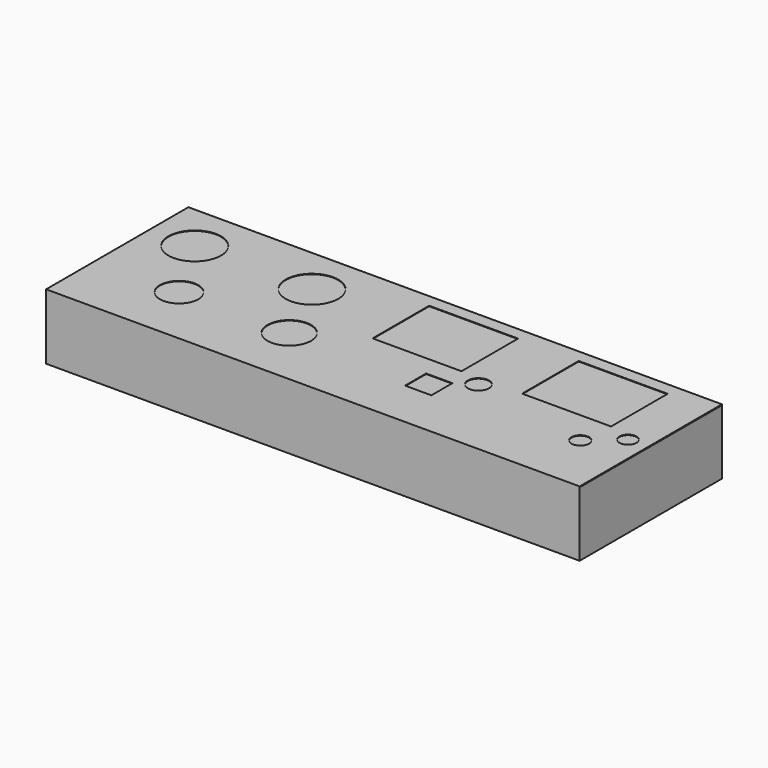
from build123d import *

# Parameters (mm, degrees)
F1_DEPTH = 209.55
F2_W     = 20.6375
F2_H     = 20.6375
F2_W_2   = 69.85
F2_H_2   = 55.5625
F3_DEPTH = 0.4064


# Not quite as in the source:
# - the dataset's text gives a spline's control points without its knots; the knots are read off the source's solid


with BuildPart() as f1:
    # F0 (on Right) → F1 (new body, symmetric)
    with BuildSketch(Plane.YZ):
        Polygon((-139.7, 0), (0, 0), (0, 50.8), (-139.2936, 50.8), (-139.2936, 51.054), (0, 51.054), (0, 51.4604), (-139.7, 51.4604), align=None)
    extrude(amount=F1_DEPTH, both=True)

    # F2 (on face) → F3 (cut, through all)
    with BuildSketch(Plane.XY.offset(51.4604)):
        with Locations((52.6280792475, -91.7013814436)):
            Rectangle(F2_W, F2_H)
        with Locations((139.9405792475, -37.7263814436)):
            Rectangle(F2_W_2, F2_H_2)
        with Locations((22.4655792475, -37.7263814436)):
            Rectangle(F2_W_2, F2_H_2)
        with BuildLine():
            add(Edge.make_bspline(
                [(-68.9765797525, -103.7685150436), (-65.8170737525, -106.9276908436), (-61.3770521525, -108.7670064436), (-56.9094207525, -108.7670064436), (-52.4415099525, -108.7670064436), (-48.0011327525, -106.9276908436), (-44.8419569525, -103.7685150436), (-41.6828065525, -100.6093646436), (-39.8437957525, -96.1693430436), (-39.8437957525, -91.7013814436), (-39.8437957525, -87.2334452436), (-41.6828065525, -82.7933728436), (-44.8419569525, -79.6342478436), (-48.0011327525, -76.4750974436), (-52.4415099525, -74.6357564436), (-56.9094207525, -74.6357564436)],
                knots=[3, 3, 3, 3, 4, 4, 4, 5, 5, 5, 6, 6, 6, 7, 7, 7, 8, 8, 8, 8], degree=3))
            add(Edge.make_bspline(
                [(-56.9094207525, -74.6357564436), (-61.3770521525, -74.6357564436), (-65.8170737525, -76.4750974436), (-68.9765797525, -79.6342478436)],
                knots=[0, 0, 0, 0, 1, 1, 1, 1], degree=3))
            add(Edge.make_bspline(
                [(-68.9765797525, -79.6342478436), (-72.1357047525, -82.7933728436), (-73.9750457525, -87.2334452436), (-73.9750457525, -91.7013814436), (-73.9750457525, -96.1693430436), (-72.1357047525, -100.6093646436), (-68.9765797525, -103.7685150436)],
                knots=[1, 1, 1, 1, 2, 2, 2, 3, 3, 3, 3], degree=3))
        make_face()
        with BuildLine():
            add(Edge.make_bspline(
                [(82.3340650475, -66.7578702436), (80.7910150475, -65.2151250436), (78.6226678475, -64.3170064436), (76.4405792475, -64.3170064436)],
                knots=[7, 7, 7, 7, 8, 8, 8, 8], degree=3))
            add(Edge.make_bspline(
                [(76.4405792475, -64.3170064436), (74.2587700475, -64.3170064436), (72.0901180475, -65.2151250436), (70.5473728475, -66.7578702436)],
                knots=[0, 0, 0, 0, 1, 1, 1, 1], degree=3))
            add(Edge.make_bspline(
                [(70.5473728475, -66.7578702436), (69.0046784475, -68.3009202436), (68.1062042475, -70.4695722436), (68.1062042475, -72.6513814436), (68.1062042475, -74.8331652436), (69.0046784475, -77.0018680436), (70.5473728475, -78.5445624436)],
                knots=[1, 1, 1, 1, 2, 2, 2, 3, 3, 3, 3], degree=3))
            add(Edge.make_bspline(
                [(70.5473728475, -78.5445624436), (72.0901180475, -80.0876124436), (74.2587700475, -80.9857564436), (76.4405792475, -80.9857564436), (78.6226678475, -80.9857564436), (80.7910150475, -80.0876124436), (82.3340650475, -78.5445624436)],
                knots=[3, 3, 3, 3, 4, 4, 4, 5, 5, 5, 5], degree=3))
            add(Edge.make_bspline(
                [(82.3340650475, -78.5445624436), (83.8771658475, -77.0018680436), (84.7749542475, -74.8331652436), (84.7749542475, -72.6513814436), (84.7749542475, -70.4695722436), (83.8771658475, -68.3009202436), (82.3340650475, -66.7578702436)],
                knots=[5, 5, 5, 5, 6, 6, 6, 7, 7, 7, 7], degree=3))
        make_face()
        with BuildLine():
            add(Edge.make_bspline(
                [(-67.7163587525, -23.1332940436), (-71.5366203525, -19.3130324436), (-76.9064851525, -17.0888814436), (-82.3094207525, -17.0888814436)],
                knots=[7, 7, 7, 7, 8, 8, 8, 8], degree=3))
            add(Edge.make_bspline(
                [(-82.3094207525, -17.0888814436), (-87.7120515525, -17.0888814436), (-93.0815607525, -19.3130324436), (-96.9021525525, -23.1332940436)],
                knots=[0, 0, 0, 0, 1, 1, 1, 1], degree=3))
            add(Edge.make_bspline(
                [(-96.9021525525, -23.1332940436), (-100.7227697525, -26.9539112436), (-102.9469207525, -32.3234458436), (-102.9469207525, -37.7263814436), (-102.9469207525, -43.1293170436), (-100.7227697525, -48.4988770436), (-96.9021525525, -52.3194434436)],
                knots=[1, 1, 1, 1, 2, 2, 2, 3, 3, 3, 3], degree=3))
            add(Edge.make_bspline(
                [(-96.9021525525, -52.3194434436), (-93.0815607525, -56.1397050436), (-87.7120515525, -58.3638814436), (-82.3094207525, -58.3638814436), (-76.9064851525, -58.3638814436), (-71.5366203525, -56.1397050436), (-67.7163587525, -52.3194434436)],
                knots=[3, 3, 3, 3, 4, 4, 4, 5, 5, 5, 5], degree=3))
            add(Edge.make_bspline(
                [(-67.7163587525, -52.3194434436), (-63.8960971525, -48.4988770436), (-61.6719207525, -43.1293170436), (-61.6719207525, -37.7263814436), (-61.6719207525, -32.3234458436), (-63.8960971525, -26.9539112436), (-67.7163587525, -23.1332940436)],
                knots=[5, 5, 5, 5, 6, 6, 6, 7, 7, 7, 7], degree=3))
        make_face()
        with BuildLine():
            add(Edge.make_bspline(
                [(-159.7913587525, -23.1332940436), (-163.6116203525, -19.3130324436), (-168.9814851525, -17.0888814436), (-174.3844207525, -17.0888814436)],
                knots=[7, 7, 7, 7, 8, 8, 8, 8], degree=3))
            add(Edge.make_bspline(
                [(-174.3844207525, -17.0888814436), (-179.7870515525, -17.0888814436), (-185.1565607525, -19.3130324436), (-188.9771525525, -23.1332940436)],
                knots=[0, 0, 0, 0, 1, 1, 1, 1], degree=3))
            add(Edge.make_bspline(
                [(-188.9771525525, -23.1332940436), (-192.7977697525, -26.9539112436), (-195.0219207525, -32.3234458436), (-195.0219207525, -37.7263814436), (-195.0219207525, -43.1293170436), (-192.7977697525, -48.4988770436), (-188.9771525525, -52.3194434436)],
                knots=[1, 1, 1, 1, 2, 2, 2, 3, 3, 3, 3], degree=3))
            add(Edge.make_bspline(
                [(-188.9771525525, -52.3194434436), (-185.1565607525, -56.1397050436), (-179.7870515525, -58.3638814436), (-174.3844207525, -58.3638814436), (-168.9814851525, -58.3638814436), (-163.6116203525, -56.1397050436), (-159.7913587525, -52.3194434436)],
                knots=[3, 3, 3, 3, 4, 4, 4, 5, 5, 5, 5], degree=3))
            add(Edge.make_bspline(
                [(-159.7913587525, -52.3194434436), (-155.9710971525, -48.4988770436), (-153.7469207525, -43.1293170436), (-153.7469207525, -37.7263814436), (-153.7469207525, -32.3234458436), (-155.9710971525, -26.9539112436), (-159.7913587525, -23.1332940436)],
                knots=[5, 5, 5, 5, 6, 6, 6, 7, 7, 7, 7], degree=3))
        make_face()
        with BuildLine():
            add(Edge.make_bspline(
                [(-132.7995407525, -81.0370644436), (-135.5914579525, -78.2455028436), (-139.5154277525, -76.6201314436), (-143.4638577525, -76.6201314436)],
                knots=[7, 7, 7, 7, 8, 8, 8, 8], degree=3))
            add(Edge.make_bspline(
                [(-143.4638577525, -76.6201314436), (-147.4119321525, -76.6201314436), (-151.3358765525, -78.2455028436), (-154.1277937525, -81.0370644436)],
                knots=[0, 0, 0, 0, 1, 1, 1, 1], degree=3))
            add(Edge.make_bspline(
                [(-154.1277937525, -81.0370644436), (-156.9197109525, -83.8290070436), (-158.5451077525, -87.7529514436), (-158.5451077525, -91.7013814436), (-158.5451077525, -95.6498114436), (-156.9197109525, -99.5737558436), (-154.1277937525, -102.3653174436)],
                knots=[1, 1, 1, 1, 2, 2, 2, 3, 3, 3, 3], degree=3))
            add(Edge.make_bspline(
                [(-154.1277937525, -102.3653174436), (-151.3358765525, -105.1572346436), (-147.4119321525, -106.7826314436), (-143.4638577525, -106.7826314436), (-139.5154277525, -106.7826314436), (-135.5914579525, -105.1572346436), (-132.7995407525, -102.3653174436), (-130.0079791525, -99.5737558436), (-128.3826077525, -95.6498114436), (-128.3826077525, -91.7013814436), (-128.3826077525, -87.7529514436), (-130.0079791525, -83.8290070436), (-132.7995407525, -81.0370644436)],
                knots=[3, 3, 3, 3, 4, 4, 4, 5, 5, 5, 6, 6, 6, 7, 7, 7, 7], degree=3))
        make_face()
        with BuildLine():
            add(Edge.make_bspline(
                [(176.6018978475, -86.7903930436), (175.3161752475, -85.5046958436), (173.5088890475, -84.7560562436), (171.6905792475, -84.7560562436)],
                knots=[7, 7, 7, 7, 8, 8, 8, 8], degree=3))
            add(Edge.make_bspline(
                [(171.6905792475, -84.7560562436), (169.8722440475, -84.7560562436), (168.0652880475, -85.5046958436), (166.7795908475, -86.7903930436)],
                knots=[0, 0, 0, 0, 1, 1, 1, 1], degree=3))
            add(Edge.make_bspline(
                [(166.7795908475, -86.7903930436), (165.4938936475, -88.0761156436), (164.7452540475, -89.8830462436), (164.7452540475, -91.7013814436), (164.7452540475, -93.5196912436), (165.4938936475, -95.3266472436), (166.7795908475, -96.6123444436)],
                knots=[1, 1, 1, 1, 2, 2, 2, 3, 3, 3, 3], degree=3))
            add(Edge.make_bspline(
                [(166.7795908475, -96.6123444436), (168.0652880475, -97.8980670436), (169.8722440475, -98.6466812436), (171.6905792475, -98.6466812436), (173.5088890475, -98.6466812436), (175.3161752475, -97.8980670436), (176.6018978475, -96.6123444436), (177.8875950475, -95.3266472436), (178.6358790475, -93.5196912436), (178.6358790475, -91.7013814436), (178.6358790475, -89.8830462436), (177.8875950475, -88.0761156436), (176.6018978475, -86.7903930436)],
                knots=[3, 3, 3, 3, 4, 4, 4, 5, 5, 5, 6, 6, 6, 7, 7, 7, 7], degree=3))
        make_face()
        with BuildLine():
            add(Edge.make_bspline(
                [(198.6863088475, -67.8806264436), (197.4374924475, -66.6317592436), (195.6822000475, -65.9045064436), (193.9155792475, -65.9045064436)],
                knots=[7, 7, 7, 7, 8, 8, 8, 8], degree=3))
            add(Edge.make_bspline(
                [(193.9155792475, -65.9045064436), (192.1492886475, -65.9045064436), (190.3939962475, -66.6317592436), (189.1447988475, -67.8806264436)],
                knots=[0, 0, 0, 0, 1, 1, 1, 1], degree=3))
            add(Edge.make_bspline(
                [(189.1447988475, -67.8806264436), (187.8959316475, -69.1294428436), (187.1687042475, -70.8850908436), (187.1687042475, -72.6513814436), (187.1687042475, -74.4176974436), (187.8959316475, -76.1732946436), (189.1447988475, -77.4221618436)],
                knots=[1, 1, 1, 1, 2, 2, 2, 3, 3, 3, 3], degree=3))
            add(Edge.make_bspline(
                [(189.1447988475, -77.4221618436), (190.3939962475, -78.6710036436), (192.1492886475, -79.3982564436), (193.9155792475, -79.3982564436), (195.6822000475, -79.3982564436), (197.4374924475, -78.6710036436), (198.6863088475, -77.4221618436)],
                knots=[3, 3, 3, 3, 4, 4, 4, 5, 5, 5, 5], degree=3))
            add(Edge.make_bspline(
                [(198.6863088475, -77.4221618436), (199.9355062475, -76.1732946436), (200.6624542475, -74.4176974436), (200.6624542475, -72.6513814436), (200.6624542475, -70.8850908436), (199.9355062475, -69.1294428436), (198.6863088475, -67.8806264436)],
                knots=[5, 5, 5, 5, 6, 6, 6, 7, 7, 7, 7], degree=3))
        make_face()
    extrude(amount=-F3_DEPTH, mode=Mode.SUBTRACT)


solid = f1.part
